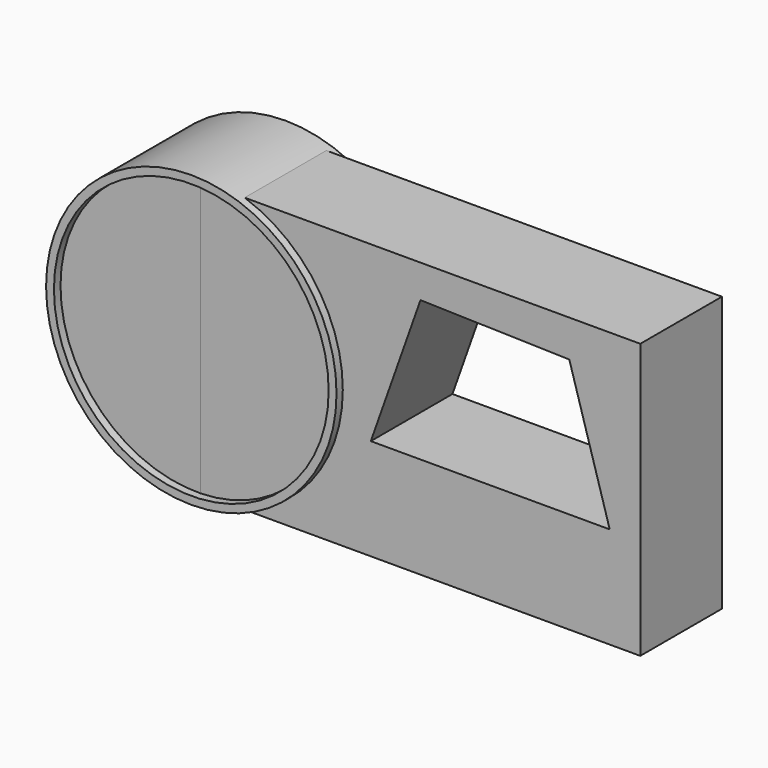
from build123d import *

# Parameters (mm, degrees)
F1_R     = 23.4951168528
F1_R_2   = 22.225
F2_DEPTH = 9.525
F0_W     = 71.12
F0_H     = 44.45
F3_DEPTH = 8.255
F5_DEPTH = 6.35
F7_DEPTH = 17.781


# Not quite as in the source:
# - the program builds the solid bodies; features that only make, move or delete a surface that nothing else refers to are left out


with BuildPart() as f2:
    # F1 (on Front) → F2 (new body, symmetric)
    with BuildSketch(Plane.XZ):
        with Locations((-36.0651165247, 0)):
            Circle(F1_R)
        with Locations((-36.0651165247, 0)):
            Circle(F1_R_2, mode=Mode.SUBTRACT)
    extrude(amount=F2_DEPTH, both=True)

    # F0 (on Front) → F3 (join, symmetric)
    with BuildSketch(Plane.XZ):
        Rectangle(F0_W, F0_H)
    extrude(amount=F3_DEPTH, both=True)

    # F6 (on face) → F7 (cut, through all)
    with BuildSketch(Plane.XZ.offset(8.255)):
        Polygon((0, 16.8832416568), (-8.0388132402, -5.8187644509), (30.6133943614, -5.8187644509), (24.0750207475, 16.2531816351), align=None)
    extrude(amount=-F7_DEPTH, mode=Mode.SUBTRACT)


with BuildPart() as f5:
    # F4 (on face) → F5 (new body)
    with BuildSketch(Plane.XZ.offset(8.255)):
        with BuildLine():
            Line((-35.56, -22.2192592653), (-35.56, 22.2192592653))
            ThreePointArc((-35.56, 22.2192592653), (-58.242372306, 0), (-35.56, -22.2192592653))
        make_face()
    extrude(amount=-F5_DEPTH)


solid = Compound([f2.part, f5.part])
